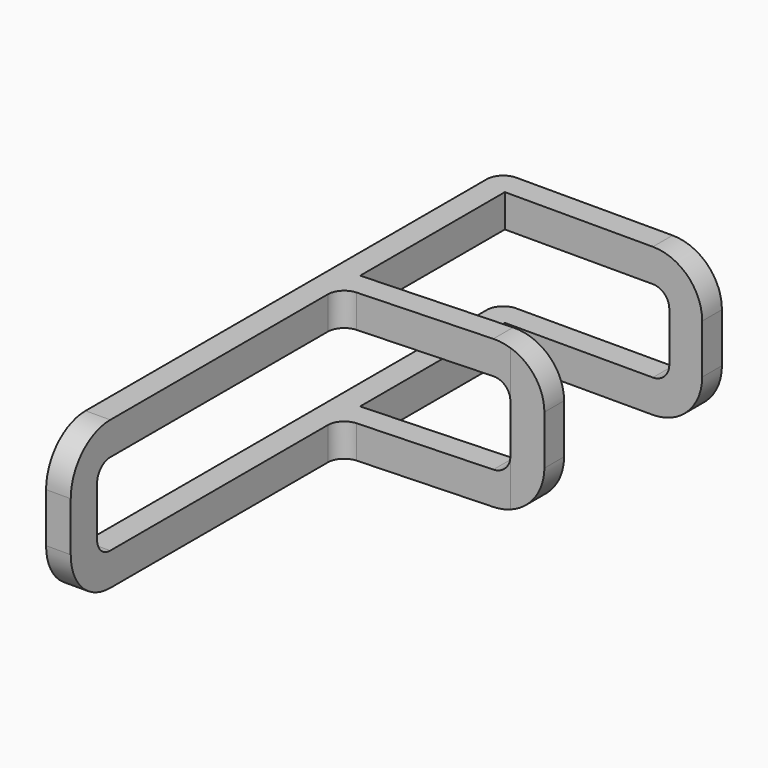
from build123d import *

# Parameters (mm, degrees)
F1_DEPTH      = 2.5
F1_DEPTH_BACK = 2.5
F2_SIZE2      = 1
F2_SIZE       = 2
F3_R          = 3
F4_START      = 4
F4_DEPTH      = 5
F5_R          = 5
F5_2_R        = 5
F6_R          = 2
F6_2_R        = 2
F7_W          = 2.5
F7_H          = 2.5
F8_ANGLE      = 90
F9_DEPTH      = 10
F11_DEPTH     = 8
F12_DEPTH     = 8
F15_START     = 2.5
F14_R         = 2.5
F15_DEPTH     = 1.5
F16_W         = 12
F16_H         = 2
F16_W_2       = 2
F16_H_2       = 20
F17_DEPTH     = 7
F18_T         = -1
F16_H_3       = 1.5
F16_W_3       = 1.5
F19_DEPTH     = 9
F20_START     = 2
F20_DEPTH     = 5
F21_R         = 3
F21_2_R       = 3
F22_T1_DEPTH  = 2
F22_T3_DEPTH  = 1
F22_T5_DEPTH  = 1
F22_T7_DEPTH  = 2
F22_T9_DEPTH  = 2
F22_T11_DEPTH = 11
F22_T13_DEPTH = 32
F22_S17_W     = 1.02
F22_S17_H     = 1.02
F22_T18_DEPTH = 1.02
F22_S23_W     = 1.02
F22_S23_H     = 1.02
F22_T24_DEPTH = 1.02
F22_T28_ANGLE = 233.2969892374
F22_T30_ANGLE = 233.2969892374
F22_T32_ANGLE = 233.2969892374
F22_T34_ANGLE = 233.2969892374
F22_T35_DEPTH = 9
F22_T37_DEPTH = 9
F22_T39_DEPTH = 17
F22_T42_ANGLE = 233.2969892374
F22_T44_ANGLE = 90
F22_T46_ANGLE = 233.2969892374
F22_T48_ANGLE = 90
F22_T50_ANGLE = 90
F22_T52_ANGLE = 233.2969892374
F22_T54_ANGLE = 233.2969892374
F22_T56_ANGLE = 90
F22_T58_ANGLE = 233.2969892374
F22_T60_ANGLE = 233.2969892374
F22_T62_ANGLE = 90
F22_T64_ANGLE = 233.2969892374
F22_T66_ANGLE = 90
F22_T68_ANGLE = 233.2969892374
F22_2_F1_R    = 1
F22_2_F2_R    = 1


# Not quite as in the source:
# - a fillet or chamfer that OpenCascade refuses, or shapes differently, is made with other operations: its cross-section is extruded or revolved along the edge and cut away or added
# - a feature names something its author has since deleted; it is built from what else it names


with BuildPart() as f1:
    # F0 (on Top) → F1 (new body, two sides)
    with BuildSketch(Plane.XY) as f1_sk:
        Polygon((-2.4175545031, 19.9997189244), (-63.6058346017, 10), (-71.3429901912, 55.5274909482), (-73.2526121256, 67.2124675644), (-87.2356820635, 67.2124675644), (-132.104240014, 0), (-120.0807613656, 0), (-81.7352983314, 57.4409632971), (-81.1490054203, 53.9442313206), (-72.104240014, 0), (-63.6058346017, 0), (-0.7575159774, 9.8419431859), (0.8509074882, 0), (10.9835668635, 0), (4.4465969461, 39.9997189244), (-5.6860624292, 39.9997189244), align=None)
    extrude(amount=F1_DEPTH)
    extrude(f1_sk.sketch, amount=-F1_DEPTH_BACK)

    # F2
    f2_edges = [f1.edges().sort_by_distance(p)[0] for p in [
        (-80.244147, 67.212468, 2.5),
    ]]
    f2_side = f1.faces().sort_by_distance((-80.244147, 67.212468, 0))[0]
    chamfer(f2_edges, length=F2_SIZE, length2=F2_SIZE2, reference=f2_side)

    # F3
    f3_edges = [f1.edges().sort_by_distance(p)[0] for p in [
        (-80.496216, 66.212468, 2.5),
    ]]
    fillet(f3_edges, radius=F3_R)

    # F5
    f5_edges = [f1.edges().sort_by_distance(p)[0] for p in [
        (-81.735298, 57.440963, 0),
        (-72.10424, 0, 0),
        (-120.080761, 0, 0),
        (0.850907, 0, 0),
        (-87.235682, 67.212468, -1),
        (-73.252612, 67.212468, -1),
        (4.446597, 39.999719, 0),
    ]]
    fillet(f5_edges, radius=F5_R)

    # F6
    f6_edges = [f1.edges().sort_by_distance(p)[0] for p in [
        (-2.417555, 19.999719, 0),
        (-63.605835, 10, 0),
        (-0.757516, 9.841943, 0),
        (-5.686062, 39.999719, 0),
        (10.983567, 0, 0),
        (-132.10424, 0, 0),
    ]]
    fillet(f6_edges, radius=F6_R)

    # F7 (on Top) → F8 (revolve, cut)
    with BuildSketch(Plane.XY):
        Polygon((-82.9107738397, 68.988720722), (-82.9107738397, 65.988720722), (-82.0857738397, 65.988720722), (-79.9107738397, 65.988720722), (-77.7357738397, 65.988720722), (-76.9107738397, 65.988720722), (-76.9107738397, 68.988720722), align=None)
        Polygon((-82.4107738397, 65.488720722), (-79.9107738397, 65.488720722), (-77.4107738397, 65.488720722), (-76.9107738397, 65.1856904189), (-76.9107738397, 65.488720722), (-77.7357738397, 65.988720722), (-79.9107738397, 65.988720722), (-82.0857738397, 65.988720722), (-82.9107738397, 65.488720722), (-82.9107738397, 65.1856904189), align=None)
        Polygon((-82.9107738397, 65.988720722), (-82.9107738397, 65.488720722), (-82.0857738397, 65.988720722), align=None)
        Polygon((-77.7357738397, 65.988720722), (-76.9107738397, 65.488720722), (-76.9107738397, 65.988720722), align=None)
        Polygon((-82.9107738397, 65.1856904189), (-82.9107738397, 62.988720722), (-82.4107738397, 62.988720722), (-82.4107738397, 65.488720722), align=None)
        with Locations((-81.1607738397, 64.238720722)):
            Rectangle(F7_W, F7_H)
        with Locations((-78.6607738397, 64.238720722)):
            Rectangle(F7_W, F7_H)
        Polygon((-77.4107738397, 62.988720722), (-76.9107738397, 62.988720722), (-76.9107738397, 65.1856904189), (-77.4107738397, 65.488720722), align=None)
    revolve(axis=Axis((-79.9107738397, 62.988720722, 0), (-1, 0, 0)), revolution_arc=F8_ANGLE, mode=Mode.SUBTRACT)


with BuildPart() as f4:
    # F0 (on Top) → F4 (new body)
    with BuildSketch(Plane.XY.offset(F4_START)):
        Polygon((-2.4175545031, 19.9997189244), (-63.6058346017, 10), (-71.3429901912, 55.5274909482), (-73.2526121256, 67.2124675644), (-87.2356820635, 67.2124675644), (-132.104240014, 0), (-120.0807613656, 0), (-81.7352983314, 57.4409632971), (-81.1490054203, 53.9442313206), (-72.104240014, 0), (-63.6058346017, 0), (-0.7575159774, 9.8419431859), (0.8509074882, 0), (10.9835668635, 0), (4.4465969461, 39.9997189244), (-5.6860624292, 39.9997189244), align=None)
    extrude(amount=F4_DEPTH)

    # F5#2
    f5_2_edges = [f4.edges().sort_by_distance(p)[0] for p in [
        (-81.735298, 57.440963, 6.5),
        (-72.10424, 0, 6.5),
        (-120.080761, 0, 6.5),
        (0.850907, 0, 6.5),
        (-87.235682, 67.212468, 6.5),
        (-73.252612, 67.212468, 6.5),
        (4.446597, 39.999719, 6.5),
    ]]
    fillet(f5_2_edges, radius=F5_2_R)

    # F6#2
    f6_2_edges = [f4.edges().sort_by_distance(p)[0] for p in [
        (-2.417555, 19.999719, 6.5),
        (-63.605835, 10, 6.5),
        (-0.757516, 9.841943, 6.5),
        (-5.686062, 39.999719, 6.5),
        (10.983567, 0, 6.5),
        (-132.10424, 0, 6.5),
    ]]
    fillet(f6_2_edges, radius=F6_2_R)


with BuildPart() as f9_tool:
    # F7 (on Top) → F9 (new body)
    with BuildSketch(Plane.XY):
        Polygon((-82.9107738397, 68.988720722), (-82.9107738397, 65.988720722), (-82.0857738397, 65.988720722), (-79.9107738397, 65.988720722), (-77.7357738397, 65.988720722), (-76.9107738397, 65.988720722), (-76.9107738397, 68.988720722), align=None)
        Polygon((-82.9107738397, 65.988720722), (-82.9107738397, 65.488720722), (-82.0857738397, 65.988720722), align=None)
        Polygon((-77.7357738397, 65.988720722), (-76.9107738397, 65.488720722), (-76.9107738397, 65.988720722), align=None)
        Polygon((-82.4107738397, 65.488720722), (-79.9107738397, 65.488720722), (-77.4107738397, 65.488720722), (-76.9107738397, 65.1856904189), (-76.9107738397, 65.488720722), (-77.7357738397, 65.988720722), (-79.9107738397, 65.988720722), (-82.0857738397, 65.988720722), (-82.9107738397, 65.488720722), (-82.9107738397, 65.1856904189), align=None)
        Polygon((-82.9107738397, 65.1856904189), (-82.9107738397, 62.988720722), (-82.4107738397, 62.988720722), (-82.4107738397, 65.488720722), align=None)
        with Locations((-81.1607738397, 64.238720722)):
            Rectangle(F7_W, F7_H)
        with Locations((-78.6607738397, 64.238720722)):
            Rectangle(F7_W, F7_H)
        Polygon((-77.4107738397, 62.988720722), (-76.9107738397, 62.988720722), (-76.9107738397, 65.1856904189), (-77.4107738397, 65.488720722), align=None)
        Polygon((-82.9107738397, 59.988720722), (-79.9107738397, 59.988720722), (-79.9107738397, 60.488720722), (-82.4107738397, 60.488720722), (-82.4107738397, 62.988720722), (-82.9107738397, 62.988720722), align=None)
        with Locations((-81.1607738397, 61.738720722)):
            Rectangle(F7_W, F7_H)
        with Locations((-78.6607738397, 61.738720722)):
            Rectangle(F7_W, F7_H)
        Polygon((-79.9107738397, 60.488720722), (-79.9107738397, 59.988720722), (-76.9107738397, 59.988720722), (-76.9107738397, 62.988720722), (-77.4107738397, 62.988720722), (-77.4107738397, 60.488720722), align=None)
    extrude(amount=F9_DEPTH)


with BuildPart() as f1_1:
    add(f1.part)

    # F9: cut by f9_tool
    add(f9_tool.part, mode=Mode.SUBTRACT)

    # F7 (on Top) → F10 (revolve, cut)
    with BuildSketch(Plane.XY):
        Polygon((-85.7107738397, 63.488720722), (-82.9107738397, 65.1856904189), (-82.9107738397, 65.488720722), (-86.2107738397, 63.488720722), (-86.2107738397, 62.988720722), (-85.7107738397, 62.988720722), align=None)
        Polygon((-85.7107738397, 62.988720722), (-82.9107738397, 62.988720722), (-82.9107738397, 65.1856904189), (-85.7107738397, 63.488720722), align=None)
        Polygon((-82.4107738397, 65.488720722), (-79.9107738397, 65.488720722), (-77.4107738397, 65.488720722), (-76.9107738397, 65.1856904189), (-76.9107738397, 65.488720722), (-77.7357738397, 65.988720722), (-79.9107738397, 65.988720722), (-82.0857738397, 65.988720722), (-82.9107738397, 65.488720722), (-82.9107738397, 65.1856904189), align=None)
        Polygon((-82.9107738397, 65.1856904189), (-82.9107738397, 62.988720722), (-82.4107738397, 62.988720722), (-82.4107738397, 65.488720722), align=None)
        with Locations((-81.1607738397, 64.238720722)):
            Rectangle(F7_W, F7_H)
        with Locations((-78.6607738397, 64.238720722)):
            Rectangle(F7_W, F7_H)
        Polygon((-77.4107738397, 62.988720722), (-76.9107738397, 62.988720722), (-76.9107738397, 65.1856904189), (-77.4107738397, 65.488720722), align=None)
        Polygon((-76.9107738397, 65.1856904189), (-76.9107738397, 62.988720722), (-74.1107738397, 62.988720722), (-74.1107738397, 63.488720722), align=None)
        Polygon((-76.9107738397, 65.488720722), (-76.9107738397, 65.1856904189), (-74.1107738397, 63.488720722), (-74.1107738397, 62.988720722), (-73.6107738397, 62.988720722), (-73.6107738397, 63.488720722), align=None)
    revolve(axis=Axis((-75.7607738397, 62.988720722, 0), (1, 0, 0)), mode=Mode.SUBTRACT)

    # F7 (on Top) → F11 (cut)
    with BuildSketch(Plane.XY):
        with Locations((-78.6607738397, 64.238720722)):
            Rectangle(F7_W, F7_H)
        with Locations((-81.1607738397, 64.238720722)):
            Rectangle(F7_W, F7_H)
        with Locations((-78.6607738397, 61.738720722)):
            Rectangle(F7_W, F7_H)
        with Locations((-81.1607738397, 61.738720722)):
            Rectangle(F7_W, F7_H)
    extrude(amount=F11_DEPTH, mode=Mode.SUBTRACT)



with BuildPart() as f4_1:
    add(f4.part)

    # F9: cut by f9_tool
    add(f9_tool.part, mode=Mode.SUBTRACT)


with BuildPart() as f12:
    # F7 (on Top) → F12 (new body)
    with BuildSketch(Plane.XY):
        with Locations((-81.1607738397, 64.238720722)):
            Rectangle(F7_W, F7_H)
        with Locations((-78.6607738397, 64.238720722)):
            Rectangle(F7_W, F7_H)
        with Locations((-81.1607738397, 61.738720722)):
            Rectangle(F7_W, F7_H)
        with Locations((-78.6607738397, 61.738720722)):
            Rectangle(F7_W, F7_H)
    extrude(amount=F12_DEPTH)

    # F7 (on Top) → F13 (revolve)
    with BuildSketch(Plane.XY):
        Polygon((-85.7107738397, 62.988720722), (-82.9107738397, 62.988720722), (-82.9107738397, 65.1856904189), (-85.7107738397, 63.488720722), align=None)
        Polygon((-82.9107738397, 65.1856904189), (-82.9107738397, 62.988720722), (-82.4107738397, 62.988720722), (-82.4107738397, 65.488720722), align=None)
        with Locations((-81.1607738397, 64.238720722)):
            Rectangle(F7_W, F7_H)
        with Locations((-78.6607738397, 64.238720722)):
            Rectangle(F7_W, F7_H)
        Polygon((-77.4107738397, 62.988720722), (-76.9107738397, 62.988720722), (-76.9107738397, 65.1856904189), (-77.4107738397, 65.488720722), align=None)
        Polygon((-76.9107738397, 65.1856904189), (-76.9107738397, 62.988720722), (-74.1107738397, 62.988720722), (-74.1107738397, 63.488720722), align=None)
    revolve(axis=Axis((-79.9107738397, 62.988720722, 0), (1, 0, 0)))


with BuildPart() as f1_2:
    add(f1_1.part)

    add(f4_1.part)  # F15 merges F4
    # F14 (on Top) → F15 (join)
    with BuildSketch(Plane.XY.offset(F15_START)):
        with Locations((5.1001101943, 5)):
            Circle(F14_R)
        with Locations((0.6434008568, 34.9997189244)):
            Circle(F14_R)
        with Locations((-122.7546855807, 5)):
            Circle(F14_R)
        with Locations((-67.8727891486, 5)):
            Circle(F14_R)
        with Locations((-81.4505400433, 54.6900098794)):
            Circle(F14_R)
    extrude(amount=F15_DEPTH)


with BuildPart() as f17:
    # F16 (on Top) → F17 (new body)
    with BuildSketch(Plane.XY):
        Polygon((-30.1369051993, -11.2915403917), (-30.1369051993, -0.2915403917), (-18.1369051993, -0.2915403917), (-18.1369051993, 1.7084596083), (-32.1369051993, 1.7084596083), (-32.1369051993, -13.2915403917), (-30.1369051993, -13.2915403917), align=None)
        with Locations((-24.1369051993, -12.2915403917)):
            Rectangle(F16_W, F16_H)
        with Locations((-31.1369051993, -23.2915403917)):
            Rectangle(F16_W_2, F16_H_2)
    extrude(amount=F17_DEPTH)

    # F18
    f18_openings = [f17.faces().sort_by_distance(p)[0] for p in [
        (-30.136905, -23.29154, 3.5),
        (-30.136905, -5.79154, 3.5),
        (-24.136905, -13.29154, 3.5),
        (-24.136905, -0.29154, 3.5),
        (-24.136905, -11.29154, 3.5),
        (-25.136905, 1.70846, 3.5),
        (-32.136905, -15.79154, 3.5),
    ]]
    offset(amount=F18_T, openings=f18_openings)

    # F21
    f21_edges = [f17.edges().sort_by_distance(p)[0] for p in [
        (-31.136905, -33.29154, 7),
        (-31.136905, -33.29154, 0),
        (-18.136905, -12.29154, 0),
        (-18.136905, -12.29154, 7),
        (-18.136905, 0.70846, 7),
        (-18.136905, 0.70846, 0),
    ]]
    fillet(f21_edges, radius=F21_R)

    # F22: fillet of radius 1 on 28 edges, made by hand

    # F22_s2 → F22_t1 (join)
    with BuildSketch(Plane.YZ.offset(-32.1369051993)):
        with BuildLine():
            ThreePointArc((-31.2915403917, 1), (-31.9986471729, 1.2928932188), (-32.2915403917, 2))
            Line((-32.2915403917, 2), (-32.3115403917, 2))
            Line((-32.3115403917, 2), (-32.3115403917, 0.98))
            Line((-32.3115403917, 0.98), (-31.2915403917, 0.98))
            Line((-31.2915403917, 0.98), (-31.2915403917, 1))
        make_face()
        with BuildLine():
            ThreePointArc((-31.2915403917, 6), (-31.9986471729, 5.7071067812), (-32.2915403917, 5))
            Line((-32.2915403917, 5), (-32.3115403917, 5))
            Line((-32.3115403917, 5), (-32.3115403917, 6.02))
            Line((-32.3115403917, 6.02), (-31.2915403917, 6.02))
            Line((-31.2915403917, 6.02), (-31.2915403917, 6))
        make_face()
    extrude(amount=F22_T1_DEPTH)

    # F22_s4 → F22_t3 (join)
    with BuildSketch(Plane.XY):
        with BuildLine():
            ThreePointArc((-29.1369051993, -0.2915403917), (-29.8440119805, -0.5844336106), (-30.1369051993, -1.2915403917))
            Line((-30.1369051993, -1.2915403917), (-30.1569051993, -1.2915403917))
            Line((-30.1569051993, -1.2915403917), (-30.1569051993, -0.2715403917))
            Line((-30.1569051993, -0.2715403917), (-29.1369051993, -0.2715403917))
            Line((-29.1369051993, -0.2715403917), (-29.1369051993, -0.2915403917))
        make_face()
        with BuildLine():
            ThreePointArc((-29.1369051993, -13.2915403917), (-29.8440119805, -13.5844336106), (-30.1369051993, -14.2915403917))
            Line((-30.1369051993, -14.2915403917), (-30.1569051993, -14.2915403917))
            Line((-30.1569051993, -14.2915403917), (-30.1569051993, -13.2715403917))
            Line((-30.1569051993, -13.2715403917), (-29.1369051993, -13.2715403917))
            Line((-29.1369051993, -13.2715403917), (-29.1369051993, -13.2915403917))
        make_face()
        with BuildLine():
            ThreePointArc((-30.1369051993, -10.2915403917), (-29.8440119805, -10.9986471729), (-29.1369051993, -11.2915403917))
            Line((-29.1369051993, -11.2915403917), (-29.1369051993, -11.3115403917))
            Line((-29.1369051993, -11.3115403917), (-30.1569051993, -11.3115403917))
            Line((-30.1569051993, -11.3115403917), (-30.1569051993, -10.2915403917))
            Line((-30.1569051993, -10.2915403917), (-30.1369051993, -10.2915403917))
        make_face()
    extrude(amount=F22_T3_DEPTH)

    # F22_s6 → F22_t5 (join)
    with BuildSketch(Plane.XY.offset(6)):
        with BuildLine():
            ThreePointArc((-29.1369051993, -0.2915403917), (-29.8440119805, -0.5844336106), (-30.1369051993, -1.2915403917))
            Line((-30.1369051993, -1.2915403917), (-30.1569051993, -1.2915403917))
            Line((-30.1569051993, -1.2915403917), (-30.1569051993, -0.2715403917))
            Line((-30.1569051993, -0.2715403917), (-29.1369051993, -0.2715403917))
            Line((-29.1369051993, -0.2715403917), (-29.1369051993, -0.2915403917))
        make_face()
        with BuildLine():
            ThreePointArc((-29.1369051993, -13.2915403917), (-29.8440119805, -13.5844336106), (-30.1369051993, -14.2915403917))
            Line((-30.1369051993, -14.2915403917), (-30.1569051993, -14.2915403917))
            Line((-30.1569051993, -14.2915403917), (-30.1569051993, -13.2715403917))
            Line((-30.1569051993, -13.2715403917), (-29.1369051993, -13.2715403917))
            Line((-29.1369051993, -13.2715403917), (-29.1369051993, -13.2915403917))
        make_face()
        with BuildLine():
            ThreePointArc((-30.1369051993, -10.2915403917), (-29.8440119805, -10.9986471729), (-29.1369051993, -11.2915403917))
            Line((-29.1369051993, -11.2915403917), (-29.1369051993, -11.3115403917))
            Line((-29.1369051993, -11.3115403917), (-30.1569051993, -11.3115403917))
            Line((-30.1569051993, -11.3115403917), (-30.1569051993, -10.2915403917))
            Line((-30.1569051993, -10.2915403917), (-30.1369051993, -10.2915403917))
        make_face()
    extrude(amount=F22_T5_DEPTH)

    # F22_s8 → F22_t7 (join)
    with BuildSketch(Plane.XZ.offset(-1.7084596083)):
        with BuildLine():
            ThreePointArc((-20.1369051993, 1), (-19.4297984181, 1.2928932188), (-19.1369051993, 2))
            Line((-19.1369051993, 2), (-19.1169051993, 2))
            Line((-19.1169051993, 2), (-19.1169051993, 0.98))
            Line((-19.1169051993, 0.98), (-20.1369051993, 0.98))
            Line((-20.1369051993, 0.98), (-20.1369051993, 1))
        make_face()
        with BuildLine():
            ThreePointArc((-20.1369051993, 6), (-19.4297984181, 5.7071067812), (-19.1369051993, 5))
            Line((-19.1369051993, 5), (-19.1169051993, 5))
            Line((-19.1169051993, 5), (-19.1169051993, 6.02))
            Line((-19.1169051993, 6.02), (-20.1369051993, 6.02))
            Line((-20.1369051993, 6.02), (-20.1369051993, 6))
        make_face()
    extrude(amount=F22_T7_DEPTH)

    # F22_s10 → F22_t9 (join)
    with BuildSketch(Plane.XZ.offset(11.2915403917)):
        with BuildLine():
            ThreePointArc((-20.1369051993, 1), (-19.4297984181, 1.2928932188), (-19.1369051993, 2))
            Line((-19.1369051993, 2), (-19.1169051993, 2))
            Line((-19.1169051993, 2), (-19.1169051993, 0.98))
            Line((-19.1169051993, 0.98), (-20.1369051993, 0.98))
            Line((-20.1369051993, 0.98), (-20.1369051993, 1))
        make_face()
        with BuildLine():
            ThreePointArc((-20.1369051993, 6), (-19.4297984181, 5.7071067812), (-19.1369051993, 5))
            Line((-19.1369051993, 5), (-19.1169051993, 5))
            Line((-19.1169051993, 5), (-19.1169051993, 6.02))
            Line((-19.1169051993, 6.02), (-20.1369051993, 6.02))
            Line((-20.1369051993, 6.02), (-20.1369051993, 6))
        make_face()
    extrude(amount=F22_T9_DEPTH)

    # F22_s12 → F22_t11 (cut)
    with BuildSketch(Plane.YZ.offset(-31.1369051993)):
        with BuildLine():
            ThreePointArc((1.7084596083, 0), (1.4155663894, 0.7071067812), (0.7084596083, 1))
            Line((0.7084596083, 1), (0.7084596083, 1.02))
            Line((0.7084596083, 1.02), (1.7284596083, 1.02))
            Line((1.7284596083, 1.02), (1.7284596083, 0))
            Line((1.7284596083, 0), (1.7084596083, 0))
        make_face()
        with BuildLine():
            ThreePointArc((1.7084596083, 7), (1.4155663894, 6.2928932188), (0.7084596083, 6))
            Line((0.7084596083, 6), (0.7084596083, 5.98))
            Line((0.7084596083, 5.98), (1.7284596083, 5.98))
            Line((1.7284596083, 5.98), (1.7284596083, 7))
            Line((1.7284596083, 7), (1.7084596083, 7))
        make_face()
    extrude(amount=F22_T11_DEPTH, mode=Mode.SUBTRACT)

    # F22_s14 → F22_t13 (cut)
    with BuildSketch(Plane.XZ.offset(-0.7084596083)):
        with BuildLine():
            ThreePointArc((-31.1369051993, 1), (-31.8440119805, 0.7071067812), (-32.1369051993, 0))
            Line((-32.1369051993, 0), (-32.1569051993, 0))
            Line((-32.1569051993, 0), (-32.1569051993, 1.02))
            Line((-32.1569051993, 1.02), (-31.1369051993, 1.02))
            Line((-31.1369051993, 1.02), (-31.1369051993, 1))
        make_face()
        with BuildLine():
            ThreePointArc((-31.1369051993, 6), (-31.8440119805, 6.2928932188), (-32.1369051993, 7))
            Line((-32.1369051993, 7), (-32.1569051993, 7))
            Line((-32.1569051993, 7), (-32.1569051993, 5.98))
            Line((-32.1569051993, 5.98), (-31.1369051993, 5.98))
            Line((-31.1369051993, 5.98), (-31.1369051993, 6))
        make_face()
    extrude(amount=F22_T13_DEPTH, mode=Mode.SUBTRACT)


with BuildPart() as f19:
    # F16 (on Top) → F19 (new body)
    with BuildSketch(Plane.XY):
        Polygon((1.4721279692, -11.7915420532), (1.4721279692, -0.7915420532), (11.4721279692, -0.7915420532), (11.4721279692, 0.7084579468), (-0.0278720308, 0.7084579468), (-0.0278720308, -31.7915420532), (1.4721279692, -31.7915420532), (1.4721279692, -13.2928435719), align=None)
        with Locations((12.4721279692, -0.0415420532)):
            Rectangle(F16_W_2, F16_H_3)
        with Locations((0.7221279692, -32.7915420532)):
            Rectangle(F16_W_3, F16_H)
        Polygon((11.4721279692, -11.3748753866), (1.4721279692, -11.7915420532), (1.4721279692, -13.2928435719), (11.4721279692, -12.8761769052), align=None)
        Polygon((13.4721279692, -11.2915420532), (11.4721279692, -11.3748753866), (11.4721279692, -12.8761769052), (13.4721279692, -12.7928435719), (13.4721279692, -11.7915420532), align=None)
    extrude(amount=F19_DEPTH)


with BuildPart() as f20_tool:
    # F16 (on Top) → F20 (new body)
    with BuildSketch(Plane.XY.offset(F20_START)):
        Polygon((1.4721279692, -11.7915420532), (1.4721279692, -0.7915420532), (11.4721279692, -0.7915420532), (11.4721279692, 0.7084579468), (-0.0278720308, 0.7084579468), (-0.0278720308, -31.7915420532), (1.4721279692, -31.7915420532), (1.4721279692, -13.2928435719), align=None)
        Polygon((11.4721279692, -11.3748753866), (1.4721279692, -11.7915420532), (1.4721279692, -13.2928435719), (11.4721279692, -12.8761769052), align=None)
    extrude(amount=F20_DEPTH)


with BuildPart() as f1_3:
    add(f1_2.part)

    # F20: cut by f20_tool
    add(f20_tool.part, mode=Mode.SUBTRACT)


with BuildPart() as f19_1:
    add(f19.part)

    # F20: cut by f20_tool
    add(f20_tool.part, mode=Mode.SUBTRACT)

    # F21#2
    f21_2_edges = [f19_1.edges().sort_by_distance(p)[0] for p in [
        (0.722128, -33.791542, 9),
        (0.722128, -33.791542, 0),
        (13.472128, -12.042193, 9),
        (13.472128, -0.041542, 9),
        (13.472128, -0.041542, 0),
        (13.472128, -12.042193, 0),
    ]]
    fillet(f21_2_edges, radius=F21_2_R)

    # F22#2: fillet of radius 1 on 10 edges, made by hand

    # F22_2_f1
    f22_2_f1_edges = [f19_1.edges().sort_by_distance(p)[0] for p in [
        (0.7221279692, -31.7915420532, 2),
        (0.7221279692, -31.7915420532, 7),
        (11.4721279692, -0.0415420532, 2),
        (11.4721279692, -0.0415420532, 7),
        (11.4721279692, -12.1255261459, 2),
        (11.4721279692, -12.1255261459, 7),
        (1.4721279692, -13.2928435719, 1),
        (1.4721279692, -13.2928435719, 8),
    ]]
    fillet(f22_2_f1_edges, radius=F22_2_F1_R)

    # F22_2_f2
    f22_2_f2_edges = [f19_1.edges().sort_by_distance(p)[0] for p in [
        (-0.0278720308, 0.7084579468, 1),
        (-0.0278720308, 0.7084579468, 8),
    ]]
    fillet(f22_2_f2_edges, radius=F22_2_F2_R)


with BuildPart() as f22_tool16:
    # F22_s17 → F22_t18 (new body)
    with BuildSketch(Plane.XY):
        with Locations((-31.6469051993, 1.2184596083)):
            Rectangle(F22_S17_W, F22_S17_H)
    extrude(amount=F22_T18_DEPTH)

    # F22_s19 → F22_t20 (revolve, cut)
    with BuildSketch(Plane(origin=(-31.1369051993, 0.7084596083, 0), x_dir=(0.7071067812, -0.7071067812, 0), z_dir=(-0.7071067812, -0.7071067812, 0))):
        with BuildLine():
            ThreePointArc((0, -1), (1, 0), (0, 1))
            Line((0, 1), (0, -1))
        make_face()
    revolve(axis=Axis((-31.1369051993, 0.7084596083, 0), (0, 0, 1)), mode=Mode.SUBTRACT)


with BuildPart() as f17_1:
    add(f17.part)

    # F22_t15: cut F22_tool16
    add(f22_tool16.part, mode=Mode.SUBTRACT)


with BuildPart() as f22_tool22:
    # F22_s23 → F22_t24 (new body)
    with BuildSketch(Plane.XZ.offset(-0.7084596083)):
        with Locations((-31.6469051993, 6.49)):
            Rectangle(F22_S23_W, F22_S23_H)
    extrude(amount=-F22_T24_DEPTH)

    # F22_s25 → F22_t26 (revolve, cut)
    with BuildSketch(Plane(origin=(-31.1369051993, 0.7084596083, 7), x_dir=(0.7071067812, 0, 0.7071067812), z_dir=(-0.7071067812, 0, 0.7071067812))):
        with BuildLine():
            ThreePointArc((0, -1), (1, 0), (0, 1))
            Line((0, 1), (0, -1))
        make_face()
    revolve(axis=Axis((-31.1369051993, 0.7084596083, 7), (0, 1, 0)), mode=Mode.SUBTRACT)


with BuildPart() as f17_2:
    add(f17_1.part)

    # F22_t21: cut F22_tool22
    add(f22_tool22.part, mode=Mode.SUBTRACT)

    # F22_s27 → F22_t28 (revolve, cut)
    with BuildSketch(Plane.XZ.offset(31.2915403917)):
        with BuildLine():
            ThreePointArc((-32.1369051993, 7), (-31.8440119805, 6.2928932188), (-31.1369051993, 6))
            Line((-31.1369051993, 6), (-31.1369051993, 5.98))
            Line((-31.1369051993, 5.98), (-32.1569051993, 5.98))
            Line((-32.1569051993, 5.98), (-32.1569051993, 7))
            Line((-32.1569051993, 7), (-32.1369051993, 7))
        make_face()
    revolve(axis=Axis((-32.1369051993, -31.2915403917, 5), (1, 0, 0)), revolution_arc=F22_T28_ANGLE, mode=Mode.SUBTRACT)

    # F22_s29 → F22_t30 (revolve, cut)
    with BuildSketch(Plane.YZ.offset(-20.1369051993)):
        with BuildLine():
            ThreePointArc((1.7084596083, 7), (1.4155663894, 6.2928932188), (0.7084596083, 6))
            Line((0.7084596083, 6), (0.7084596083, 5.98))
            Line((0.7084596083, 5.98), (1.7284596083, 5.98))
            Line((1.7284596083, 5.98), (1.7284596083, 7))
            Line((1.7284596083, 7), (1.7084596083, 7))
        make_face()
    revolve(axis=Axis((-20.1369051993, 1.7084596083, 5), (0, 1, 0)), revolution_arc=F22_T30_ANGLE, mode=Mode.SUBTRACT)

    # F22_s31 → F22_t32 (revolve, cut)
    with BuildSketch(Plane.XZ.offset(31.2915403917)):
        with BuildLine():
            ThreePointArc((-32.1369051993, 0), (-31.8440119805, 0.7071067812), (-31.1369051993, 1))
            Line((-31.1369051993, 1), (-31.1369051993, 1.02))
            Line((-31.1369051993, 1.02), (-32.1569051993, 1.02))
            Line((-32.1569051993, 1.02), (-32.1569051993, 0))
            Line((-32.1569051993, 0), (-32.1369051993, 0))
        make_face()
    revolve(axis=Axis((-32.1369051993, -31.2915403917, 2), (-1, 0, 0)), revolution_arc=F22_T32_ANGLE, mode=Mode.SUBTRACT)

    # F22_s33 → F22_t34 (revolve, cut)
    with BuildSketch(Plane.YZ.offset(-20.1369051993)):
        with BuildLine():
            ThreePointArc((1.7084596083, 0), (1.4155663894, 0.7071067812), (0.7084596083, 1))
            Line((0.7084596083, 1), (0.7084596083, 1.02))
            Line((0.7084596083, 1.02), (1.7284596083, 1.02))
            Line((1.7284596083, 1.02), (1.7284596083, 0))
            Line((1.7284596083, 0), (1.7084596083, 0))
        make_face()
    revolve(axis=Axis((-20.1369051993, 1.7084596083, 2), (0, -1, 0)), revolution_arc=F22_T34_ANGLE, mode=Mode.SUBTRACT)

    # F22_s36 → F22_t35 (cut)
    with BuildSketch(Plane.XZ.offset(1.2915403917)):
        with BuildLine():
            ThreePointArc((-31.1369051993, 1), (-30.4297984181, 0.7071067812), (-30.1369051993, 0))
            Line((-30.1369051993, 0), (-30.1169051993, 0))
            Line((-30.1169051993, 0), (-30.1169051993, 1.02))
            Line((-30.1169051993, 1.02), (-31.1369051993, 1.02))
            Line((-31.1369051993, 1.02), (-31.1369051993, 1))
        make_face()
        with BuildLine():
            ThreePointArc((-31.1369051993, 6), (-30.4297984181, 6.2928932188), (-30.1369051993, 7))
            Line((-30.1369051993, 7), (-30.1169051993, 7))
            Line((-30.1169051993, 7), (-30.1169051993, 5.98))
            Line((-30.1169051993, 5.98), (-31.1369051993, 5.98))
            Line((-31.1369051993, 5.98), (-31.1369051993, 6))
        make_face()
    extrude(amount=F22_T35_DEPTH, mode=Mode.SUBTRACT)

    # F22_s38 → F22_t37 (cut)
    with BuildSketch(Plane.YZ.offset(-29.1369051993)):
        with BuildLine():
            ThreePointArc((-0.2915403917, 0), (0.0013528271, 0.7071067812), (0.7084596083, 1))
            Line((0.7084596083, 1), (0.7084596083, 1.02))
            Line((0.7084596083, 1.02), (-0.3115403917, 1.02))
            Line((-0.3115403917, 1.02), (-0.3115403917, 0))
            Line((-0.3115403917, 0), (-0.2915403917, 0))
        make_face()
        with BuildLine():
            ThreePointArc((-0.2915403917, 7), (0.0013528271, 6.2928932188), (0.7084596083, 6))
            Line((0.7084596083, 6), (0.7084596083, 5.98))
            Line((0.7084596083, 5.98), (-0.3115403917, 5.98))
            Line((-0.3115403917, 5.98), (-0.3115403917, 7))
            Line((-0.3115403917, 7), (-0.2915403917, 7))
        make_face()
        with BuildLine():
            ThreePointArc((-12.2915403917, 1), (-12.9986471729, 0.7071067812), (-13.2915403917, 0))
            Line((-13.2915403917, 0), (-13.3115403917, 0))
            Line((-13.3115403917, 0), (-13.3115403917, 1.02))
            Line((-13.3115403917, 1.02), (-12.2915403917, 1.02))
            Line((-12.2915403917, 1.02), (-12.2915403917, 1))
        make_face()
        with BuildLine():
            ThreePointArc((-12.2915403917, 6), (-12.9986471729, 6.2928932188), (-13.2915403917, 7))
            Line((-13.2915403917, 7), (-13.3115403917, 7))
            Line((-13.3115403917, 7), (-13.3115403917, 5.98))
            Line((-13.3115403917, 5.98), (-12.2915403917, 5.98))
            Line((-12.2915403917, 5.98), (-12.2915403917, 6))
        make_face()
        with BuildLine():
            ThreePointArc((-12.2915403917, 1), (-11.5844336106, 0.7071067812), (-11.2915403917, 0))
            Line((-11.2915403917, 0), (-11.2715403917, 0))
            Line((-11.2715403917, 0), (-11.2715403917, 1.02))
            Line((-11.2715403917, 1.02), (-12.2915403917, 1.02))
            Line((-12.2915403917, 1.02), (-12.2915403917, 1))
        make_face()
        with BuildLine():
            ThreePointArc((-12.2915403917, 6), (-11.5844336106, 6.2928932188), (-11.2915403917, 7))
            Line((-11.2915403917, 7), (-11.2715403917, 7))
            Line((-11.2715403917, 7), (-11.2715403917, 5.98))
            Line((-11.2715403917, 5.98), (-12.2915403917, 5.98))
            Line((-12.2915403917, 5.98), (-12.2915403917, 6))
        make_face()
    extrude(amount=F22_T37_DEPTH, mode=Mode.SUBTRACT)

    # F22_s40 → F22_t39 (cut)
    with BuildSketch(Plane.XZ.offset(14.2915403917)):
        with BuildLine():
            ThreePointArc((-31.1369051993, 1), (-30.4297984181, 0.7071067812), (-30.1369051993, 0))
            Line((-30.1369051993, 0), (-30.1169051993, 0))
            Line((-30.1169051993, 0), (-30.1169051993, 1.02))
            Line((-30.1169051993, 1.02), (-31.1369051993, 1.02))
            Line((-31.1369051993, 1.02), (-31.1369051993, 1))
        make_face()
        with BuildLine():
            ThreePointArc((-31.1369051993, 6), (-30.4297984181, 6.2928932188), (-30.1369051993, 7))
            Line((-30.1369051993, 7), (-30.1169051993, 7))
            Line((-30.1169051993, 7), (-30.1169051993, 5.98))
            Line((-30.1169051993, 5.98), (-31.1369051993, 5.98))
            Line((-31.1369051993, 5.98), (-31.1369051993, 6))
        make_face()
    extrude(amount=F22_T39_DEPTH, mode=Mode.SUBTRACT)

    # F22_s41 → F22_t42 (revolve, cut)
    with BuildSketch(Plane.YZ.offset(-20.1369051993)):
        with BuildLine():
            ThreePointArc((-11.2915403917, 7), (-11.5844336106, 6.2928932188), (-12.2915403917, 6))
            Line((-12.2915403917, 6), (-12.2915403917, 5.98))
            Line((-12.2915403917, 5.98), (-11.2715403917, 5.98))
            Line((-11.2715403917, 5.98), (-11.2715403917, 7))
            Line((-11.2715403917, 7), (-11.2915403917, 7))
        make_face()
    revolve(axis=Axis((-20.1369051993, -11.2915403917, 5), (0, 1, 0)), revolution_arc=F22_T42_ANGLE, mode=Mode.SUBTRACT)

    # F22_s43 → F22_t44 (revolve, cut)
    with BuildSketch(Plane.XZ.offset(10.2915403917)):
        with BuildLine():
            ThreePointArc((-31.1369051993, 6), (-30.4297984181, 6.2928932188), (-30.1369051993, 7))
            Line((-30.1369051993, 7), (-30.1169051993, 7))
            Line((-30.1169051993, 7), (-30.1169051993, 5.98))
            Line((-30.1169051993, 5.98), (-31.1369051993, 5.98))
            Line((-31.1369051993, 5.98), (-31.1369051993, 6))
        make_face()
    revolve(axis=Axis((-29.1369051993, -10.2915403917, 6), (0, 0, 1)), revolution_arc=F22_T44_ANGLE, mode=Mode.SUBTRACT)

    # F22_s45 → F22_t46 (revolve, cut)
    with BuildSketch(Plane.YZ.offset(-20.1369051993)):
        with BuildLine():
            ThreePointArc((-11.2915403917, 0), (-11.5844336106, 0.7071067812), (-12.2915403917, 1))
            Line((-12.2915403917, 1), (-12.2915403917, 1.02))
            Line((-12.2915403917, 1.02), (-11.2715403917, 1.02))
            Line((-11.2715403917, 1.02), (-11.2715403917, 0))
            Line((-11.2715403917, 0), (-11.2915403917, 0))
        make_face()
    revolve(axis=Axis((-20.1369051993, -11.2915403917, 2), (0, -1, 0)), revolution_arc=F22_T46_ANGLE, mode=Mode.SUBTRACT)

    # F22_s47 → F22_t48 (revolve, cut)
    with BuildSketch(Plane.XZ.offset(10.2915403917)):
        with BuildLine():
            ThreePointArc((-31.1369051993, 1), (-30.4297984181, 0.7071067812), (-30.1369051993, 0))
            Line((-30.1369051993, 0), (-30.1169051993, 0))
            Line((-30.1169051993, 0), (-30.1169051993, 1.02))
            Line((-30.1169051993, 1.02), (-31.1369051993, 1.02))
            Line((-31.1369051993, 1.02), (-31.1369051993, 1))
        make_face()
    revolve(axis=Axis((-29.1369051993, -10.2915403917, 1), (0, 0, 1)), revolution_arc=F22_T48_ANGLE, mode=Mode.SUBTRACT)

    # F22_s49 → F22_t50 (revolve, cut)
    with BuildSketch(Plane.YZ.offset(-29.1369051993)):
        with BuildLine():
            ThreePointArc((-12.2915403917, 6), (-12.9986471729, 6.2928932188), (-13.2915403917, 7))
            Line((-13.2915403917, 7), (-13.3115403917, 7))
            Line((-13.3115403917, 7), (-13.3115403917, 5.98))
            Line((-13.3115403917, 5.98), (-12.2915403917, 5.98))
            Line((-12.2915403917, 5.98), (-12.2915403917, 6))
        make_face()
    revolve(axis=Axis((-29.1369051993, -14.2915403917, 6), (0, 0, 1)), revolution_arc=F22_T50_ANGLE, mode=Mode.SUBTRACT)

    # F22_s51 → F22_t52 (revolve, cut)
    with BuildSketch(Plane.YZ.offset(-20.1369051993)):
        with BuildLine():
            ThreePointArc((-13.2915403917, 7), (-12.9986471729, 6.2928932188), (-12.2915403917, 6))
            Line((-12.2915403917, 6), (-12.2915403917, 5.98))
            Line((-12.2915403917, 5.98), (-13.3115403917, 5.98))
            Line((-13.3115403917, 5.98), (-13.3115403917, 7))
            Line((-13.3115403917, 7), (-13.2915403917, 7))
        make_face()
    revolve(axis=Axis((-20.1369051993, -13.2915403917, 5), (0, 1, 0)), revolution_arc=F22_T52_ANGLE, mode=Mode.SUBTRACT)

    # F22_s53 → F22_t54 (revolve, cut)
    with BuildSketch(Plane.XZ.offset(31.2915403917)):
        with BuildLine():
            ThreePointArc((-30.1369051993, 7), (-30.4297984181, 6.2928932188), (-31.1369051993, 6))
            Line((-31.1369051993, 6), (-31.1369051993, 5.98))
            Line((-31.1369051993, 5.98), (-30.1169051993, 5.98))
            Line((-30.1169051993, 5.98), (-30.1169051993, 7))
            Line((-30.1169051993, 7), (-30.1369051993, 7))
        make_face()
    revolve(axis=Axis((-30.1369051993, -31.2915403917, 5), (1, 0, 0)), revolution_arc=F22_T54_ANGLE, mode=Mode.SUBTRACT)

    # F22_s55 → F22_t56 (revolve, cut)
    with BuildSketch(Plane.YZ.offset(-29.1369051993)):
        with BuildLine():
            ThreePointArc((-12.2915403917, 1), (-12.9986471729, 0.7071067812), (-13.2915403917, 0))
            Line((-13.2915403917, 0), (-13.3115403917, 0))
            Line((-13.3115403917, 0), (-13.3115403917, 1.02))
            Line((-13.3115403917, 1.02), (-12.2915403917, 1.02))
            Line((-12.2915403917, 1.02), (-12.2915403917, 1))
        make_face()
    revolve(axis=Axis((-29.1369051993, -14.2915403917, 1), (0, 0, 1)), revolution_arc=F22_T56_ANGLE, mode=Mode.SUBTRACT)

    # F22_s57 → F22_t58 (revolve, cut)
    with BuildSketch(Plane.YZ.offset(-20.1369051993)):
        with BuildLine():
            ThreePointArc((-13.2915403917, 0), (-12.9986471729, 0.7071067812), (-12.2915403917, 1))
            Line((-12.2915403917, 1), (-12.2915403917, 1.02))
            Line((-12.2915403917, 1.02), (-13.3115403917, 1.02))
            Line((-13.3115403917, 1.02), (-13.3115403917, 0))
            Line((-13.3115403917, 0), (-13.2915403917, 0))
        make_face()
    revolve(axis=Axis((-20.1369051993, -13.2915403917, 2), (0, -1, 0)), revolution_arc=F22_T58_ANGLE, mode=Mode.SUBTRACT)

    # F22_s59 → F22_t60 (revolve, cut)
    with BuildSketch(Plane.XZ.offset(31.2915403917)):
        with BuildLine():
            ThreePointArc((-30.1369051993, 0), (-30.4297984181, 0.7071067812), (-31.1369051993, 1))
            Line((-31.1369051993, 1), (-31.1369051993, 1.02))
            Line((-31.1369051993, 1.02), (-30.1169051993, 1.02))
            Line((-30.1169051993, 1.02), (-30.1169051993, 0))
            Line((-30.1169051993, 0), (-30.1369051993, 0))
        make_face()
    revolve(axis=Axis((-30.1369051993, -31.2915403917, 2), (-1, 0, 0)), revolution_arc=F22_T60_ANGLE, mode=Mode.SUBTRACT)

    # F22_s61 → F22_t62 (revolve, cut)
    with BuildSketch(Plane.YZ.offset(-29.1369051993)):
        with BuildLine():
            ThreePointArc((0.7084596083, 6), (0.0013528271, 6.2928932188), (-0.2915403917, 7))
            Line((-0.2915403917, 7), (-0.3115403917, 7))
            Line((-0.3115403917, 7), (-0.3115403917, 5.98))
            Line((-0.3115403917, 5.98), (0.7084596083, 5.98))
            Line((0.7084596083, 5.98), (0.7084596083, 6))
        make_face()
    revolve(axis=Axis((-29.1369051993, -1.2915403917, 6), (0, 0, 1)), revolution_arc=F22_T62_ANGLE, mode=Mode.SUBTRACT)

    # F22_s63 → F22_t64 (revolve, cut)
    with BuildSketch(Plane.YZ.offset(-20.1369051993)):
        with BuildLine():
            ThreePointArc((-0.2915403917, 7), (0.0013528271, 6.2928932188), (0.7084596083, 6))
            Line((0.7084596083, 6), (0.7084596083, 5.98))
            Line((0.7084596083, 5.98), (-0.3115403917, 5.98))
            Line((-0.3115403917, 5.98), (-0.3115403917, 7))
            Line((-0.3115403917, 7), (-0.2915403917, 7))
        make_face()
    revolve(axis=Axis((-20.1369051993, -0.2915403917, 5), (0, 1, 0)), revolution_arc=F22_T64_ANGLE, mode=Mode.SUBTRACT)

    # F22_s65 → F22_t66 (revolve, cut)
    with BuildSketch(Plane.YZ.offset(-29.1369051993)):
        with BuildLine():
            ThreePointArc((-0.2915403917, 0), (0.0013528271, 0.7071067812), (0.7084596083, 1))
            Line((0.7084596083, 1), (0.7084596083, 1.02))
            Line((0.7084596083, 1.02), (-0.3115403917, 1.02))
            Line((-0.3115403917, 1.02), (-0.3115403917, 0))
            Line((-0.3115403917, 0), (-0.2915403917, 0))
        make_face()
    revolve(axis=Axis((-29.1369051993, -1.2915403917, 1), (0, 0, 1)), revolution_arc=F22_T66_ANGLE, mode=Mode.SUBTRACT)

    # F22_s67 → F22_t68 (revolve, cut)
    with BuildSketch(Plane.YZ.offset(-20.1369051993)):
        with BuildLine():
            ThreePointArc((-0.2915403917, 0), (0.0013528271, 0.7071067812), (0.7084596083, 1))
            Line((0.7084596083, 1), (0.7084596083, 1.02))
            Line((0.7084596083, 1.02), (-0.3115403917, 1.02))
            Line((-0.3115403917, 1.02), (-0.3115403917, 0))
            Line((-0.3115403917, 0), (-0.2915403917, 0))
        make_face()
    revolve(axis=Axis((-20.1369051993, -0.2915403917, 2), (0, -1, 0)), revolution_arc=F22_T68_ANGLE, mode=Mode.SUBTRACT)


solid = f19_1.part
